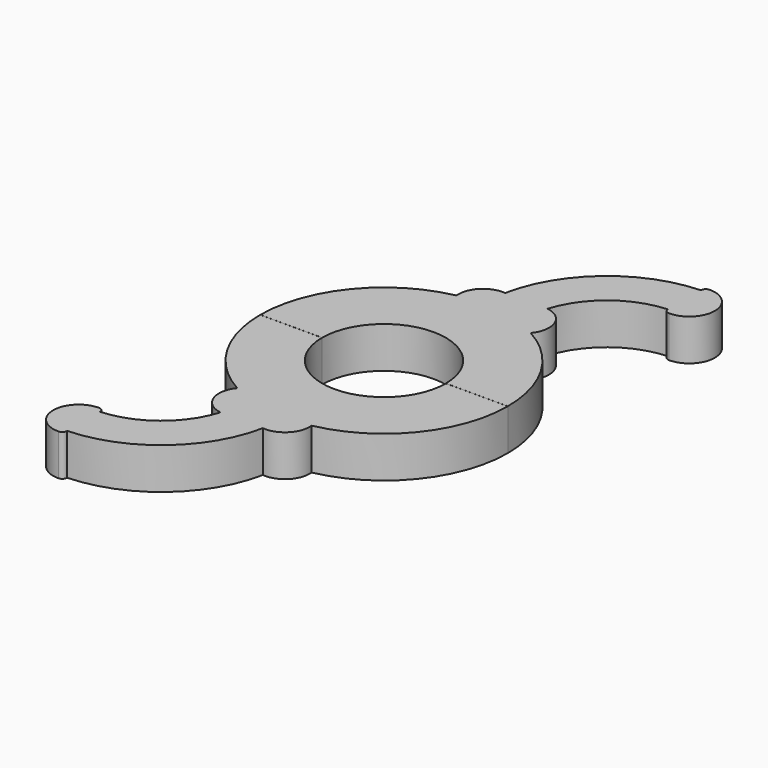
from build123d import *

# Parameters (mm, degrees)
F1_DEPTH = 10


# Not quite as in the source:
# - ends of sketch curves that miss each other by under 0.0002 mm in the source are joined


with BuildPart() as f1:
    # F0 (on Top) → F1 (new body)
    with BuildSketch(Plane.XY):
        with BuildLine():
            Line((30, 0), (15, 0))
            ThreePointArc((15, 0), (6.697e-07, -14.9804429115), (-14.9999865801, 1.75e-08))
            Line((-14.9999865801, 1.75e-08), (-30, 0))
            ThreePointArc((-30, 0), (-25.8699353497, -15.1707822858), (-14.6339808876, -26.1691157255))
            ThreePointArc((-14.6339808876, -26.1691157255), (-15.6026691532, -32.1275551224), (-10.8999993294, -35.9125588915))
            ThreePointArc((-10.8999993294, -35.9125588915), (-17.6702744626, -45.7277564826), (-28.8229878287, -49.94577897))
            ThreePointArc((-28.8229878287, -49.94577897), (-29.1797127595, -49.1356425772), (-29.9999993294, -48.8029210808))
            ThreePointArc((-29.9999993294, -48.8029210808), (-36.1775211601, -54.9804429115), (-29.9999993294, -61.1579647422))
            ThreePointArc((-29.9999993294, -61.1579647422), (-29.1592349866, -60.8048657287), (-28.8227042848, -59.9573336171))
            ThreePointArc((-28.8227042848, -59.9573336171), (-10.5622435899, -52.8315621797), (-0.5999993294, -35.9503675342))
            ThreePointArc((-0.5999993294, -35.9503675342), (4.2426413577, -34.2230835986), (5.9699252932, -29.3804429115))
            ThreePointArc((5.9699252932, -29.3804429115), (23.222002332, -18.9735637408), (30, 0))
        make_face()
    extrude(amount=F1_DEPTH)


with BuildPart() as f1b:
    # F0 (on Top) → F1, piece 2 (new body)
    with BuildSketch(Plane.XY):
        with BuildLine():
            ThreePointArc((-14.9999872507, 0.0195570727), (9e-10, 15), (14.9999872507, 0.019557071))
            Line((14.9999872507, 0.019557071), (30.0000006706, 0.0195570885))
            ThreePointArc((30.0000006706, 0.0195570885), (25.8699360203, 15.1903393743), (14.6339815581, 26.188672814))
            ThreePointArc((14.6339815581, 26.188672814), (15.6026698237, 32.1471122109), (10.9, 35.93211598))
            ThreePointArc((10.9, 35.93211598), (17.6702751331, 45.7473135711), (28.8229884993, 49.9653360585))
            ThreePointArc((28.8229884993, 49.9653360585), (29.17971343, 49.1551996657), (30, 48.8224781693))
            ThreePointArc((30, 48.8224781693), (36.1775218307, 55), (30, 61.1775218307))
            ThreePointArc((30, 61.1775218307), (29.1592356572, 60.8244228172), (28.8227049553, 59.9768907056))
            ThreePointArc((28.8227049553, 59.9768907056), (10.5622442605, 52.8511192682), (0.6, 35.9699246226))
            ThreePointArc((0.6, 35.9699246226), (-4.2426406871, 34.2426406871), (-5.9699246226, 29.4))
            ThreePointArc((-5.9699246226, 29.4), (-23.2220016615, 18.9931208293), (-29.9999936253, 0.0195570848))
            Line((-29.9999936253, 0.0195570848), (-14.9999872507, 0.0195570727))
        make_face()
    extrude(amount=F1_DEPTH)


solid = Compound([f1.part, f1b.part])
